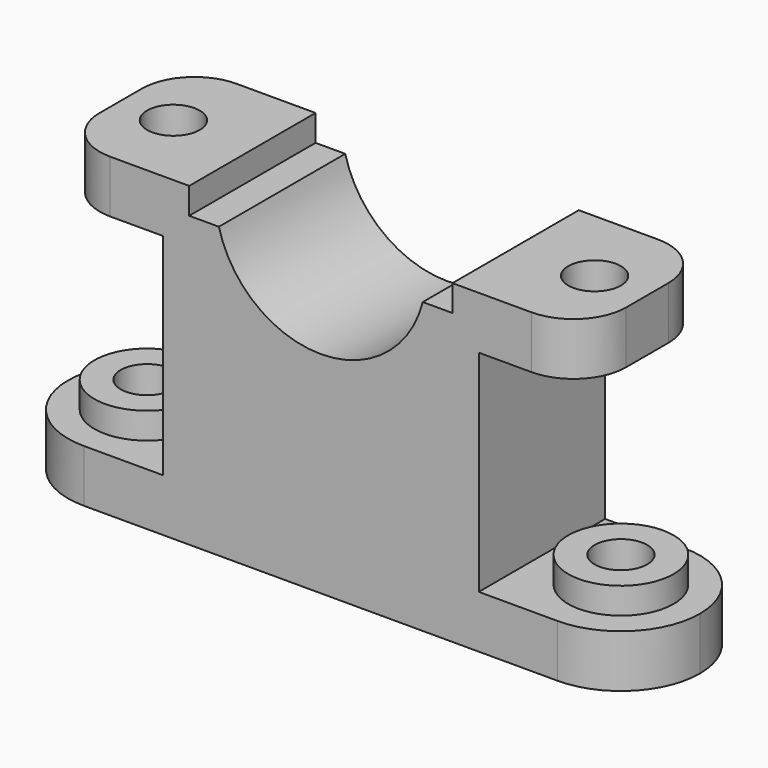
from build123d import *

# Parameters (mm, degrees)
F1_DEPTH         = 15
F2_R             = 10
F3_R             = 14.99999
F4_R             = 5
F5_DEPTH         = 10
F6_R             = 10
F7_DEPTH         = 5
F8_R             = 10
F9_DEPTH         = 5
F12_D            = 10
F12_DEPTH        = 15.001
F12_ON_F11_D     = 10
F12_ON_F11_DEPTH = 15.001


# Not quite as in the source:
# - a fillet or chamfer is up to 0.001 mm smaller than in the source, because OpenCascade refuses the exact size


with BuildPart() as f1:
    # F0 (on Front) → F1 (new body, symmetric)
    with BuildSketch(Plane.XZ):
        with BuildLine():
            Line((-60, 10), (-60, 0))
            Line((-60, 0), (60, 0))
            Line((60, 0), (60, 10))
            Line((60, 10), (30, 10))
            Line((30, 10), (30, 50))
            Line((30, 50), (50, 50))
            Line((50, 50), (50, 60))
            Line((50, 60), (25, 60))
            Line((25, 60), (25, 55))
            Line((25, 55), (19.364916731, 55))
            ThreePointArc((19.364916731, 55), (0, 40), (-19.364916731, 55))
            Line((-19.364916731, 55), (-25, 55))
            Line((-25, 55), (-25, 60))
            Line((-25, 60), (-50, 60))
            Line((-50, 60), (-50, 50))
            Line((-50, 50), (-30, 50))
            Line((-30, 50), (-30, 10))
            Line((-30, 10), (-60, 10))
        make_face()
    extrude(amount=F1_DEPTH, both=True)

    # F2
    f2_edges = [f1.edges().sort_by_distance(p)[0] for p in [
        (-50, -15, 55),
        (50, -15, 55),
        (50, 15, 55),
        (-50, 15, 55),
    ]]
    fillet(f2_edges, radius=F2_R)

    # F3 (radius 15 in the source; OpenCascade refuses exactly that, so slightly less here)
    f3_edges = [f1.edges().sort_by_distance(p)[0] for p in [
        (60, 15, 5),
        (-60, 15, 5),
        (-60, -15, 5),
        (60, -15, 5),
    ]]
    fillet(f3_edges, radius=F3_R)

    # F4 (on face) → F5 (cut, through all)
    with BuildSketch(Plane.XY.offset(60)):
        with Locations((40, 0)):
            Circle(F4_R)
        with Locations((-40, 0)):
            Circle(F4_R)
    extrude(amount=-F5_DEPTH, mode=Mode.SUBTRACT)

    # F6 (on face) → F7 (join)
    with BuildSketch(Plane.XY.offset(10)):
        with Locations((45, 0)):
            Circle(F6_R)
    extrude(amount=F7_DEPTH)

    # F8 (on face) → F9 (join)
    with BuildSketch(Plane.XY.offset(10)):
        with Locations((-45, 0)):
            Circle(F8_R)
    extrude(amount=F9_DEPTH)

    # F12 (through all, one way)
    with BuildSketch(Plane.XY.offset(15)):
        with Locations((-45, 0)):
            Circle(F12_D / 2)
    extrude(amount=-F12_DEPTH, mode=Mode.SUBTRACT)

    # F12 on F11 (through all, one way)
    with BuildSketch(Plane.XY.offset(15)):
        with Locations((45, 0)):
            Circle(F12_ON_F11_D / 2)
    extrude(amount=-F12_ON_F11_DEPTH, mode=Mode.SUBTRACT)


solid = f1.part
